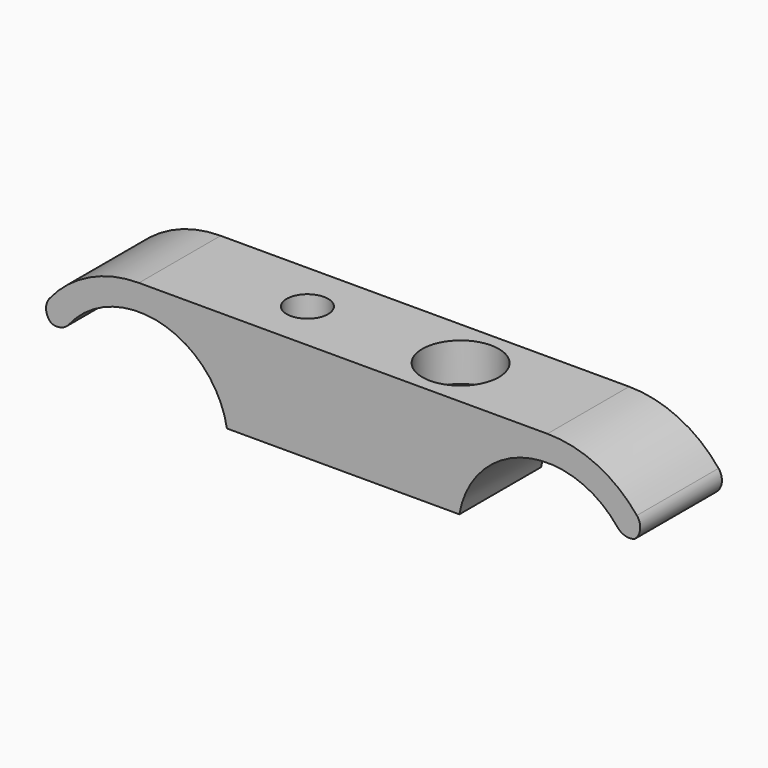
from build123d import *

# Parameters (mm, degrees)
F1_DEPTH    = 12.7
F2_R        = 3.175
F2_R_2      = 2.5796875
F3_DEPTH    = 14.2885
F2_R_3      = 4.7625
F4_DEPTH    = 4.7625
F7_T1_DEPTH = 23.7232420224
F7_T3_DEPTH = 21.5242768354
F8_W        = 32.2767272592
F8_H        = 15.9856376707
F9_DEPTH    = 1.905


# Not quite as in the source:
# - a fillet or chamfer that OpenCascade refuses, or shapes differently, is made with other operations: its cross-section is extruded or revolved along the edge and cut away or added


with BuildPart() as f1:
    # F0 (on Front) → F1 (new body)
    with BuildSketch(Plane.XZ):
        with BuildLine():
            ThreePointArc((-35.0237072996, 5.55625), (-22.5238733613, 10.7338507446), (-14.2875, 0))
            Line((-14.2875, 0), (0, 0))
            Line((0, 0), (14.2875, 0))
            ThreePointArc((14.2875, 0), (22.5238733613, 10.7338507446), (35.0237072996, 5.55625))
            Line((35.0237072996, 5.55625), (37.7733379566, 7.14375))
            ThreePointArc((37.7733379566, 7.14375), (32.54375, 12.3733379566), (25.4, 14.2875))
            Line((25.4, 14.2875), (0, 14.2875))
            Line((0, 14.2875), (-25.4, 14.2875))
            ThreePointArc((-25.4, 14.2875), (-32.54375, 12.3733379566), (-37.7733379566, 7.14375))
            Line((-37.7733379566, 7.14375), (-35.0237072996, 5.55625))
        make_face()
    extrude(amount=F1_DEPTH)

    # F2 (on face) → F3 (cut, through all)
    with BuildSketch(Plane.XY.offset(14.2875)):
        with Locations((9.525, -6.35)):
            Circle(F2_R)
        with Locations((-9.525, -6.35)):
            Circle(F2_R_2)
    extrude(amount=-F3_DEPTH, mode=Mode.SUBTRACT)

    # F2 (on face) → F4 (cut)
    with BuildSketch(Plane.XY.offset(14.2875)):
        with Locations((9.525, -6.35)):
            Circle(F2_R_3)
        with Locations((9.525, -6.35)):
            Circle(F2_R, mode=Mode.SUBTRACT)
    extrude(amount=-F4_DEPTH, mode=Mode.SUBTRACT)

    # F7: fillet of radius 1.905 on 4 edges, made by hand

    # F7_s2 → F7_t1 (cut)
    with BuildSketch(Plane.XZ.offset(-5.5116210112)):
        with BuildLine():
            ThreePointArc((-35.9958935884, 6.1175420156), (-36.9160377964, 7.4177082385), (-36.526992602, 8.9622927805))
            ThreePointArc((-36.526992602, 8.9622927805), (-37.1852941649, 8.0770971084), (-37.7733379566, 7.14375))
            Line((-37.7733379566, 7.14375), (-35.9958935884, 6.1175420156))
        make_face()
        with BuildLine():
            ThreePointArc((35.9958935884, 6.1175420156), (36.9160377964, 7.4177082385), (36.526992602, 8.9622927805))
            ThreePointArc((36.526992602, 8.9622927805), (37.1852941649, 8.0770971084), (37.7733379566, 7.14375))
            Line((37.7733379566, 7.14375), (35.9958935884, 6.1175420156))
        make_face()
    extrude(amount=F7_T1_DEPTH, mode=Mode.SUBTRACT)

    # F7_s4 → F7_t3 (cut)
    with BuildSketch(Plane.XZ.offset(-4.4121384177)):
        with BuildLine():
            ThreePointArc((-34.1069900207, 6.9047795786), (-35.242899906, 6.2171522544), (-36.5521168814, 6.4386776835))
            Line((-36.5521168814, 6.4386776835), (-35.0237072996, 5.55625))
            ThreePointArc((-35.0237072996, 5.55625), (-34.5901169235, 6.2473520136), (-34.1069900207, 6.9047795786))
        make_face()
        with BuildLine():
            ThreePointArc((34.1069900207, 6.9047795786), (35.242899906, 6.2171522544), (36.5521168814, 6.4386776835))
            Line((36.5521168814, 6.4386776835), (35.0237072996, 5.55625))
            ThreePointArc((35.0237072996, 5.55625), (34.5901169235, 6.2473520136), (34.1069900207, 6.9047795786))
        make_face()
    extrude(amount=F7_T3_DEPTH, mode=Mode.SUBTRACT)

    # F8 (on face) → F9 (cut)
    with BuildSketch(Plane(origin=(0, 0, 0), x_dir=(1, 0, 0), z_dir=(0, 0, -1))):
        with Locations((0, 6.0593477681)):
            Rectangle(F8_W, F8_H)
    extrude(amount=-F9_DEPTH, mode=Mode.SUBTRACT)


solid = f1.part
